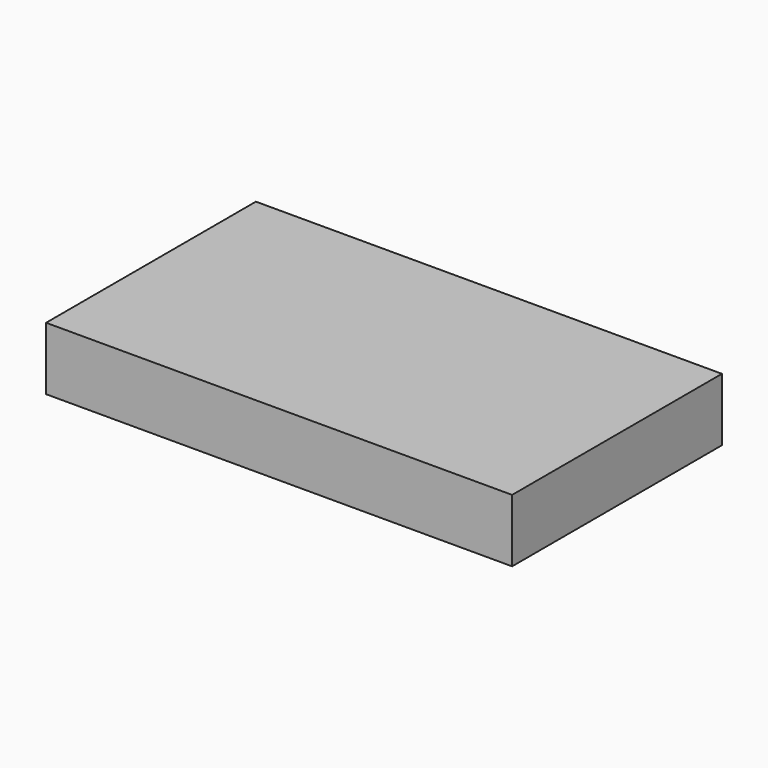
from build123d import *

# Parameters (mm, degrees)
F0_W     = 70.3723412007
F0_H     = 39.6034847945
F2_DEPTH = 9.5
F1_R     = 2.35
F3_DEPTH = 8


# Not quite as in the source:
# - the program builds the solid bodies; features that only make, move or delete a surface that nothing else refers to are left out


with BuildPart() as f2:
    # F0 (on Top) → F2 (new body)
    with BuildSketch(Plane.XY):
        with Locations((-25.7422635332, 26.3515496626)):
            Rectangle(F0_W, F0_H)
    extrude(amount=F2_DEPTH)

    # F1 (on face) → F3 (cut)
    with BuildSketch(Plane.XY):
        with BuildLine():
            ThreePointArc((-26.0081397088, 24.315958029), (-26.0169226605, 24.8283618655), (-26.0432611967, 25.3401636957))
            ThreePointArc((-26.0432611967, 25.3401636957), (-29.6543131579, 29.4708098057), (-30.4048881867, 34.9057496103))
            ThreePointArc((-30.4048881867, 34.9057496103), (-54.7680712155, 18.5828288025), (-26.0081397088, 24.315958029))
        make_face()
        with BuildLine():
            ThreePointArc((-18.4289942121, 24.2039844017), (-10.2782880331, 12.4173582289), (0.4453969671, 21.9232063115))
            ThreePointArc((0.4453969671, 21.9232063115), (0.1704350534, 24.2013451557), (-0.6386587183, 26.348642973))
            ThreePointArc((-0.6386587183, 26.348642973), (-4.6497239534, 27.6234855531), (-6.8365136406, 31.2195693659))
            ThreePointArc((-6.8365136406, 31.2195693659), (-9.2433206047, 31.4975310038), (-11.6428466394, 31.1624828835))
            ThreePointArc((-11.6428466394, 31.1624828835), (-14.0873300566, 26.758138344), (-18.4289942121, 24.2039844017))
        make_face()
        with BuildLine():
            ThreePointArc((-26.0432611967, 25.3401636957), (-22.3553467612, 23.9731105992), (-18.4289942121, 24.2039844017))
            ThreePointArc((-18.4289942121, 24.2039844017), (-15.9845107949, 28.6083289412), (-11.6428466394, 31.1624828835))
            ThreePointArc((-11.6428466394, 31.1624828835), (-11.436389736, 32.2945759735), (-11.3672378186, 33.4432609737))
            ThreePointArc((-11.3672378186, 33.4432609737), (-20.2088389756, 42.9901322485), (-30.4048881867, 34.9057496103))
            ThreePointArc((-30.4048881867, 34.9057496103), (-27.3555998695, 30.5189557333), (-26.0432611967, 25.3401636957))
        make_face()
        with Locations((-20.9422378186, 33.4432609737)):
            Circle(F1_R, mode=Mode.SUBTRACT)
        with BuildLine():
            ThreePointArc((-6.8365136406, 31.2195693659), (-3.2130730762, 29.4515061375), (-0.6386587183, 26.348642973))
            ThreePointArc((-0.6386587183, 26.348642973), (3.4064099368, 28.2070418834), (5.0577621814, 32.340958029))
            ThreePointArc((5.0577621814, 32.340958029), (-1.5054185479, 38.3144685099), (-6.8365136406, 31.2195693659))
        make_face()
        with BuildLine():
            ThreePointArc((-30.4048881867, 34.9057496103), (-29.6543131579, 29.4708098057), (-26.0432611967, 25.3401636957))
            ThreePointArc((-26.0432611967, 25.3401636957), (-27.3555998695, 30.5189557333), (-30.4048881867, 34.9057496103))
        make_face()
        with BuildLine():
            ThreePointArc((-11.6428466394, 31.1624828835), (-15.9845107949, 28.6083289412), (-18.4289942121, 24.2039844017))
            ThreePointArc((-18.4289942121, 24.2039844017), (-14.0873300566, 26.758138344), (-11.6428466394, 31.1624828835))
        make_face()
        with Locations((-20.9422378186, 33.4432609737)):
            Circle(F1_R)
        with BuildLine():
            ThreePointArc((-6.8365136406, 31.2195693659), (-4.6497239534, 27.6234855531), (-0.6386587183, 26.348642973))
            ThreePointArc((-0.6386587183, 26.348642973), (-3.2130730762, 29.4515061375), (-6.8365136406, 31.2195693659))
        make_face()
    extrude(amount=F3_DEPTH, mode=Mode.SUBTRACT)


solid = f2.part
